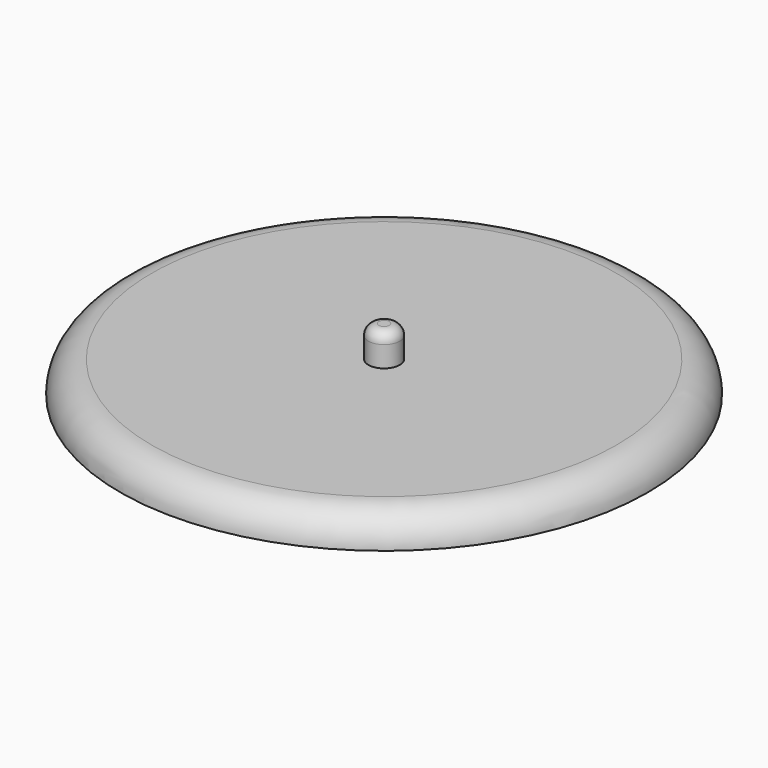
from build123d import *

# Parameters (mm, degrees)
F0_R     = 1.5
F1_DEPTH = 6
F0_R_2   = 25.2105248434
F2_DEPTH = 3
F3_R     = 1
F4_R     = 2.99999


# Not quite as in the source:
# - a fillet or chamfer is up to 0.001 mm smaller than in the source, because OpenCascade refuses the exact size
# - a feature names something its author has since deleted; it is built from what else it names


with BuildPart() as f1:
    # F0 (on Top) → F1 (new body)
    with BuildSketch(Plane.XY):
        with Locations((-25.4, 0)):
            Circle(F0_R)
    extrude(amount=F1_DEPTH)

    # F3
    f3_edges = [f1.edges().sort_by_distance(p)[0] for p in [
        (-26.9, 0, 6),
    ]]
    fillet(f3_edges, radius=F3_R)


with BuildPart() as f2:
    # F0 (on Top) → F2 (new body)
    with BuildSketch(Plane.XY):
        with Locations((-25.4, 0)):
            Circle(F0_R_2)
        with Locations((-25.4, 0)):
            Circle(F0_R, mode=Mode.SUBTRACT)
    extrude(amount=F2_DEPTH)

    # F4 (radius 3 in the source; OpenCascade refuses exactly that, so slightly less here)
    f4_edges = [f2.edges().sort_by_distance(p)[0] for p in [
        (-50.610525, 0, 3),
    ]]
    fillet(f4_edges, radius=F4_R)


solid = Compound([f1.part, f2.part])
